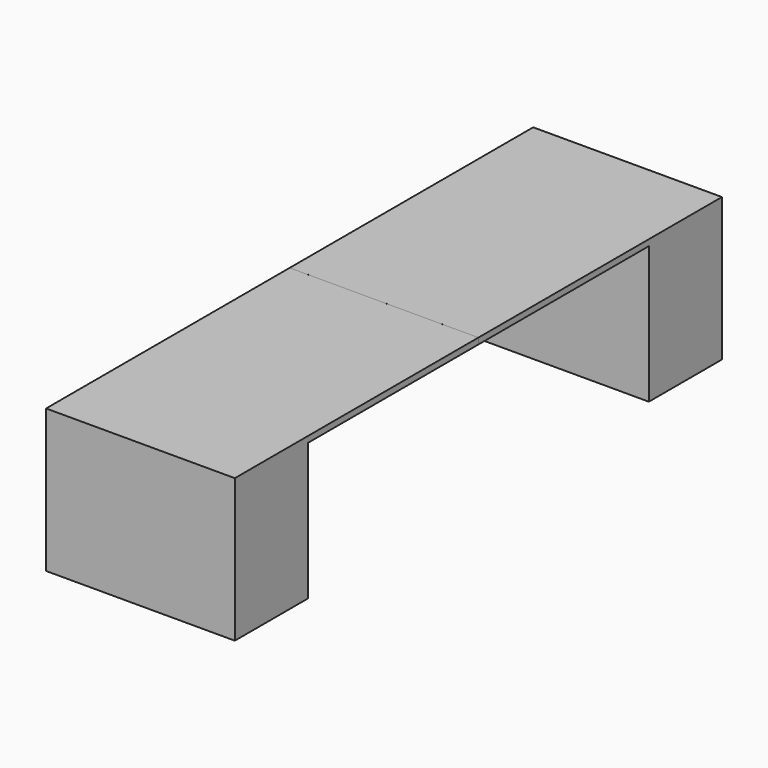
from build123d import *

# Parameters (mm, degrees)
F0_W        = 200
F0_H        = 47
F1_DEPTH    = 62
F2_W        = 140
F2_H        = 45
F3_DEPTH    = 61
F4_T        = 1
F4_T3_DEPTH = 63
F4_T5_DEPTH = 47
F4_T7_DEPTH = 142
F5_W        = 70.8849802613
F5_H        = 0.001
F6_DEPTH    = 120


# Not quite as in the source:
# - a shell that OpenCascade refuses in one call is made with other operations: the cavity is built on its own and cut out


with BuildPart() as f1:
    # F0 (on Right) → F1 (new body)
    with BuildSketch(Plane.YZ):
        with Locations((0, 23.5)):
            Rectangle(F0_W, F0_H)
    extrude(amount=-F1_DEPTH)

    # F2 (on face) → F3 (cut)
    with BuildSketch(Plane.YZ):
        with Locations((0, 22.5)):
            Rectangle(F2_W, F2_H)
    extrude(amount=-F3_DEPTH, mode=Mode.SUBTRACT)

    # F4: shell of thickness 1, made by hand


with BuildPart() as f4_core1:
    # F4_t2: copy of F1
    add(f1.part)

    # the walls: a layer under each face that stays
    f4_faces = [f4_core1.faces().sort_by_distance(p)[0] for p in [
        (-31, -100, 23.5),
        (-31, 0, 47),
        (0, -85.7142857143, 3.3571428571),
        (-62, 0, 23.5),
        (-31, 100, 23.5),
        (-30.5, -70, 22.5),
        (-61, 0, 22.5),
        (-30.5, 70, 22.5),
        (-30.5, 0, 45),
    ]]
    thicken(f4_faces, amount=-F4_T, mode=Mode.SUBTRACT)

    # F4_s4 → F4_t3 (cut)
    with BuildSketch(Plane.YZ.offset(-62)):
        Polygon((-69.99, 44.99), (-71, 45), (-71, 46), (-70, 46), align=None)
        Polygon((69.99, 44.99), (71, 45), (71, 46), (70, 46), align=None)
    extrude(amount=F4_T3_DEPTH, mode=Mode.SUBTRACT)

    # F4_s6 → F4_t5 (cut)
    with BuildSketch(Plane.XY.offset(-1)):
        Polygon((-60.99, -69.99), (-61, -71), (-62, -71), (-62, -70), align=None)
        Polygon((-60.99, 69.99), (-62, 70), (-62, 71), (-61, 71), align=None)
    extrude(amount=F4_T5_DEPTH, mode=Mode.SUBTRACT)

    # F4_s8 → F4_t7 (cut)
    with BuildSketch(Plane.XZ.offset(-71)):
        Polygon((-60.99, 44.99), (-62, 45), (-62, 46), (-61, 46), align=None)
    extrude(amount=F4_T7_DEPTH, mode=Mode.SUBTRACT)


with BuildPart() as f1_1:
    add(f1.part)

    # what is left inside the walls is the cavity
    f4_cavity = [f4_core1.part.solids().sort_by_distance(p)[0] for p in [
        (-41, -98.99, 23),
        (-41, 98.99, 23),
    ]]
    add(f4_cavity, mode=Mode.SUBTRACT)

    # F5 (on face) → F6 (cut)
    with BuildSketch(Plane(origin=(0, 0, 0), x_dir=(1, 0, 0), z_dir=(0, 0, -1))):
        with Locations((-35.4424901307, -0.0005)):
            Rectangle(F5_W, F5_H)
    extrude(amount=-F6_DEPTH, mode=Mode.SUBTRACT)


solid = f1_1.part
